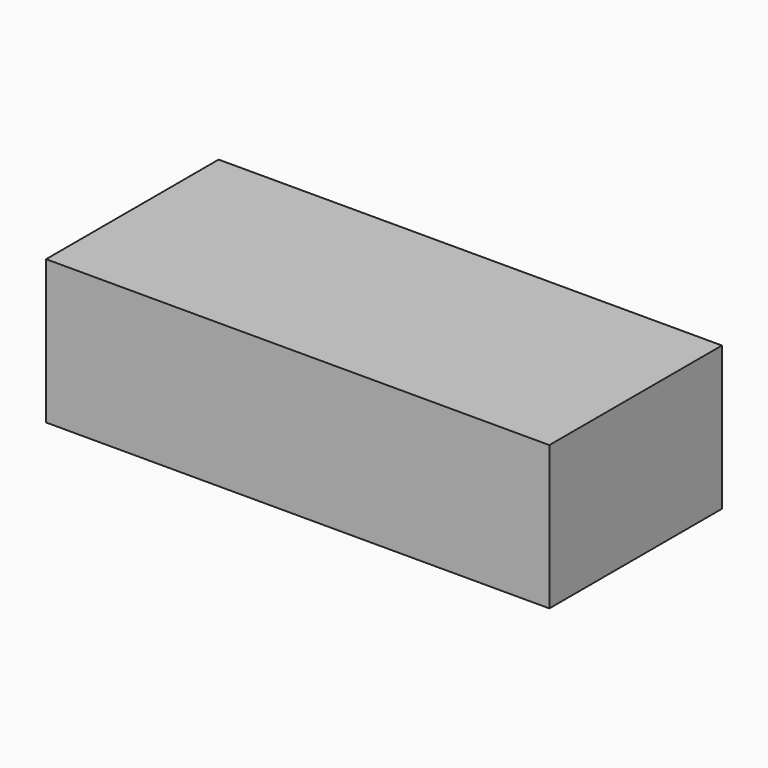
from build123d import *

# Parameters (mm, degrees)
F0_W     = 88.9
F0_H     = 38.1
F1_DEPTH = 25.4


# Not quite as in the source:
# - the program builds the solid bodies; features that only make, move or delete a surface that nothing else refers to are left out


with BuildPart() as f1:
    # F0 (on Top) → F1 (new body)
    with BuildSketch(Plane.XY):
        Rectangle(F0_W, F0_H)
    extrude(amount=F1_DEPTH)


solid = f1.part
